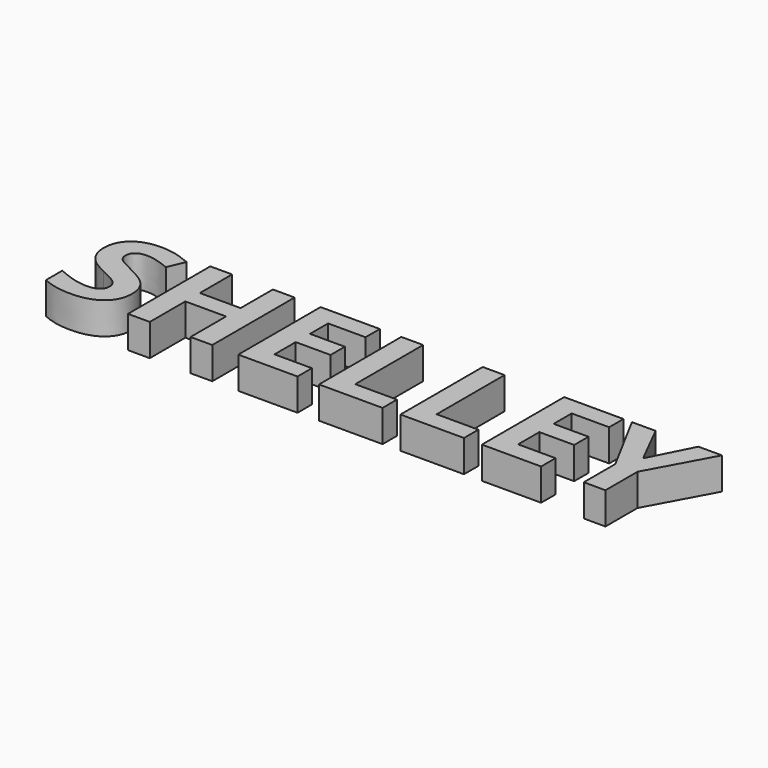
from build123d import *

# Parameters (mm, degrees)
F0_TEXT_SIZE = 9.0277777778
F1_DEPTH     = 2


# Not quite as in the source:
# - Text() gives the source's letters only with a copy of the font that has no kerning and outlines rounded to 1/6400 em; it was checked with that copy


with BuildPart() as f1:
    # F0 (on Top) → F1 (new body)
    with BuildSketch(Plane.XY):
        with Locations((-46.5330794336, -0.824576519)):
            Text('SHELLEY', F0_TEXT_SIZE, font='Open Sans', font_style=FontStyle.BOLD, text_align=(TextAlign.LEFT, TextAlign.BOTTOM))
    extrude(amount=F1_DEPTH)


solid = f1.part
